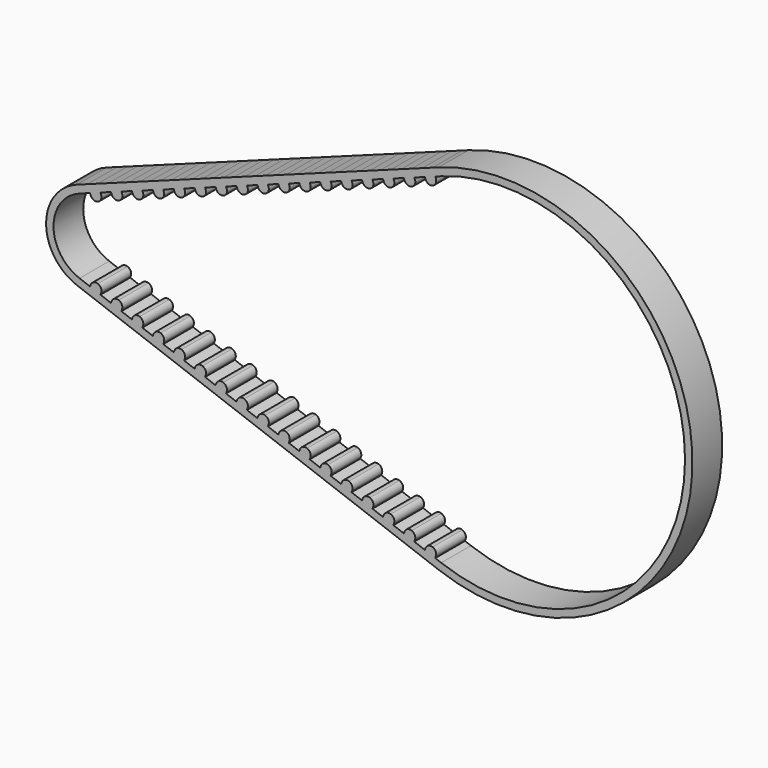
from build123d import *

# Parameters (mm, degrees)
F1_DEPTH = 10
F2_T     = -2
F3_W     = 3
F3_H     = 10
F4_DEPTH = 4
F5_R     = 1.5
F6_R     = 1.49999
F7_W     = 3
F7_H     = 10
F8_DEPTH = 4
F9_R     = 1.49999


# Not quite as in the source:
# - a fillet or chamfer is up to 0.001 mm smaller than in the source, because OpenCascade refuses the exact size


with BuildPart() as f1:
    # F0 (on Front) → F1 (new body)
    with BuildSketch(Plane.XZ):
        with BuildLine():
            Line((17.1738075313, 47.6842348629), (-80.1782614342, 11.9210587157))
            ThreePointArc((-80.1782614342, 11.9210587157), (-88.4989510894, 0), (-80.1782614342, -11.9210587157))
            Line((-80.1782614342, -11.9210587157), (17.1738075313, -47.6842348629))
            ThreePointArc((17.1738075313, -47.6842348629), (85.4910489106, 0), (17.1738075313, 47.6842348629))
        make_face()
    extrude(amount=F1_DEPTH)

    # F2
    f2_openings = [f1.faces().sort_by_distance(p)[0] for p in [
        (11.496716, -10, 0),
        (11.496716, 0, 0),
    ]]
    offset(amount=F2_T, openings=f2_openings)

    # F3 (on face) → F4 (join)
    with BuildSketch(Plane(origin=(-13.3922652901, 0, 36.4555074403), x_dir=(0.9386660406, 0, 0.3448275862), z_dir=(-0.3448275862, 0, 0.9386660406))):
        with Locations((-66.6499013013, -5)):
            Rectangle(F3_W, F3_H)
        with Locations((-60.6499013013, -5)):
            Rectangle(F3_W, F3_H)
        with Locations((-54.6499013013, -5)):
            Rectangle(F3_W, F3_H)
        with Locations((-48.6499013013, -5)):
            Rectangle(F3_W, F3_H)
        with Locations((-42.6499013013, -5)):
            Rectangle(F3_W, F3_H)
        with Locations((-36.6499013013, -5)):
            Rectangle(F3_W, F3_H)
        with Locations((-30.6499013013, -5)):
            Rectangle(F3_W, F3_H)
        with Locations((-24.6499013013, -5)):
            Rectangle(F3_W, F3_H)
        with Locations((-18.6499013013, -5)):
            Rectangle(F3_W, F3_H)
        with Locations((-12.6499013013, -5)):
            Rectangle(F3_W, F3_H)
        with Locations((-6.6499013013, -5)):
            Rectangle(F3_W, F3_H)
        with Locations((-0.6499013013, -5)):
            Rectangle(F3_W, F3_H)
        with Locations((5.3500986987, -5)):
            Rectangle(F3_W, F3_H)
        with Locations((11.3500986987, -5)):
            Rectangle(F3_W, F3_H)
        with Locations((17.3500986987, -5)):
            Rectangle(F3_W, F3_H)
        with Locations((23.3500986987, -5)):
            Rectangle(F3_W, F3_H)
        with Locations((29.3500986987, -5)):
            Rectangle(F3_W, F3_H)
    extrude(amount=-F4_DEPTH)

    # F5
    f5_edges = [f1.edges().sort_by_distance(p)[0] for p in [
        (-75.982953, -5, 9.200877),
    ]]
    fillet(f5_edges, radius=F5_R)

    # F6 (radius 1.5 in the source; OpenCascade refuses exactly that, so slightly less here)
    f6_edges = [f1.edges().sort_by_distance(p)[0] for p in [
        (-73.166955, -5, 10.23536),
        (-70.350957, -5, 11.269843),
        (-67.534959, -5, 12.304326),
        (-64.71896, -5, 13.338808),
        (-61.902962, -5, 14.373291),
        (-59.086964, -5, 15.407774),
        (-56.270966, -5, 16.442257),
        (-53.454968, -5, 17.476739),
        (-50.63897, -5, 18.511222),
        (-47.822972, -5, 19.545705),
        (-45.006974, -5, 20.580188),
        (-42.190976, -5, 21.61467),
        (-39.374977, -5, 22.649153),
        (-36.558979, -5, 23.683636),
        (-33.742981, -5, 24.718119),
        (-30.926983, -5, 25.752601),
        (-28.110985, -5, 26.787084),
        (-25.294987, -5, 27.821567),
        (-22.478989, -5, 28.85605),
        (-19.662991, -5, 29.890532),
        (-16.846992, -5, 30.925015),
        (-14.030994, -5, 31.959498),
        (-11.214996, -5, 32.993981),
        (-8.398998, -5, 34.028464),
        (-5.583, -5, 35.062946),
        (-2.767002, -5, 36.097429),
        (0.048996, -5, 37.131912),
        (2.864994, -5, 38.166395),
        (5.680993, -5, 39.200877),
        (8.496991, -5, 40.23536),
        (11.312989, -5, 41.269843),
        (14.128987, -5, 42.304326),
        (16.944985, -5, 43.338808),
    ]]
    fillet(f6_edges, radius=F6_R)

    # F7 (on face) → F8 (join)
    with BuildSketch(Plane(origin=(-13.3922652901, 0, -36.4555074403), x_dir=(0.9386660406, 0, -0.3448275862), z_dir=(-0.3448275862, 0, -0.9386660406))):
        with Locations((-66.6499013013, 5)):
            Rectangle(F7_W, F7_H)
        with Locations((-60.6499013013, 5)):
            Rectangle(F7_W, F7_H)
        with Locations((-54.6499013013, 5)):
            Rectangle(F7_W, F7_H)
        with Locations((-48.6499013013, 5)):
            Rectangle(F7_W, F7_H)
        with Locations((-42.6499013013, 5)):
            Rectangle(F7_W, F7_H)
        with Locations((-36.6499013013, 5)):
            Rectangle(F7_W, F7_H)
        with Locations((-30.6499013013, 5)):
            Rectangle(F7_W, F7_H)
        with Locations((-24.6499013013, 5)):
            Rectangle(F7_W, F7_H)
        with Locations((-18.6499013013, 5)):
            Rectangle(F7_W, F7_H)
        with Locations((-12.6499013013, 5)):
            Rectangle(F7_W, F7_H)
        with Locations((-6.6499013013, 5)):
            Rectangle(F7_W, F7_H)
        with Locations((-0.6499013013, 5)):
            Rectangle(F7_W, F7_H)
        with Locations((5.3500986987, 5)):
            Rectangle(F7_W, F7_H)
        with Locations((11.3500986987, 5)):
            Rectangle(F7_W, F7_H)
        with Locations((17.3500986987, 5)):
            Rectangle(F7_W, F7_H)
        with Locations((23.3500986987, 5)):
            Rectangle(F7_W, F7_H)
        with Locations((29.3500986987, 5)):
            Rectangle(F7_W, F7_H)
    extrude(amount=-F8_DEPTH)

    # F9 (radius 1.5 in the source; OpenCascade refuses exactly that, so slightly less here)
    f9_edges = [f1.edges().sort_by_distance(p)[0] for p in [
        (-75.982953, -5, -9.200877),
        (-73.166955, -5, -10.23536),
        (-70.350957, -5, -11.269843),
        (-67.534959, -5, -12.304326),
        (-64.71896, -5, -13.338808),
        (-59.086964, -5, -15.407774),
        (-61.902962, -5, -14.373291),
        (-56.270966, -5, -16.442257),
        (-53.454968, -5, -17.476739),
        (-50.63897, -5, -18.511222),
        (-47.822972, -5, -19.545705),
        (-45.006974, -5, -20.580188),
        (-42.190976, -5, -21.61467),
        (-39.374977, -5, -22.649153),
        (-36.558979, -5, -23.683636),
        (-33.742981, -5, -24.718119),
        (-30.926983, -5, -25.752601),
        (-28.110985, -5, -26.787084),
        (-25.294987, -5, -27.821567),
        (-22.478989, -5, -28.85605),
        (-19.662991, -5, -29.890532),
        (-16.846992, -5, -30.925015),
        (-14.030994, -5, -31.959498),
        (-11.214996, -5, -32.993981),
        (-8.398998, -5, -34.028464),
        (-5.583, -5, -35.062946),
        (-2.767002, -5, -36.097429),
        (0.048996, -5, -37.131912),
        (2.864994, -5, -38.166395),
        (5.680993, -5, -39.200877),
        (8.496991, -5, -40.23536),
        (11.312989, -5, -41.269843),
        (14.128987, -5, -42.304326),
        (16.944985, -5, -43.338808),
    ]]
    fillet(f9_edges, radius=F9_R)


solid = f1.part
